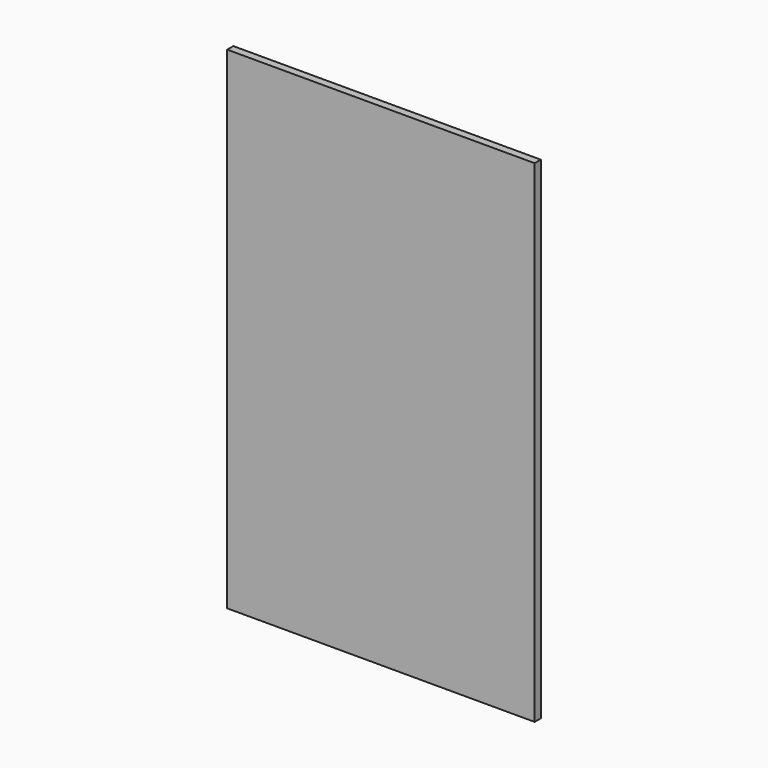
from build123d import *

# Parameters (mm, degrees)
F0_W     = 31.75
F0_H     = 50.8
F1_DEPTH = 0.79375


# Not quite as in the source:
# - a length typed as a fraction of an inch, garbled in the dataset ("3 / 203.2 mm" for 3/8 in), is restored


with BuildPart() as f1:
    # F0 (on Front) → F1 (new body)
    with BuildSketch(Plane.XZ):
        Rectangle(F0_W, F0_H)
    extrude(amount=F1_DEPTH)


solid = f1.part
